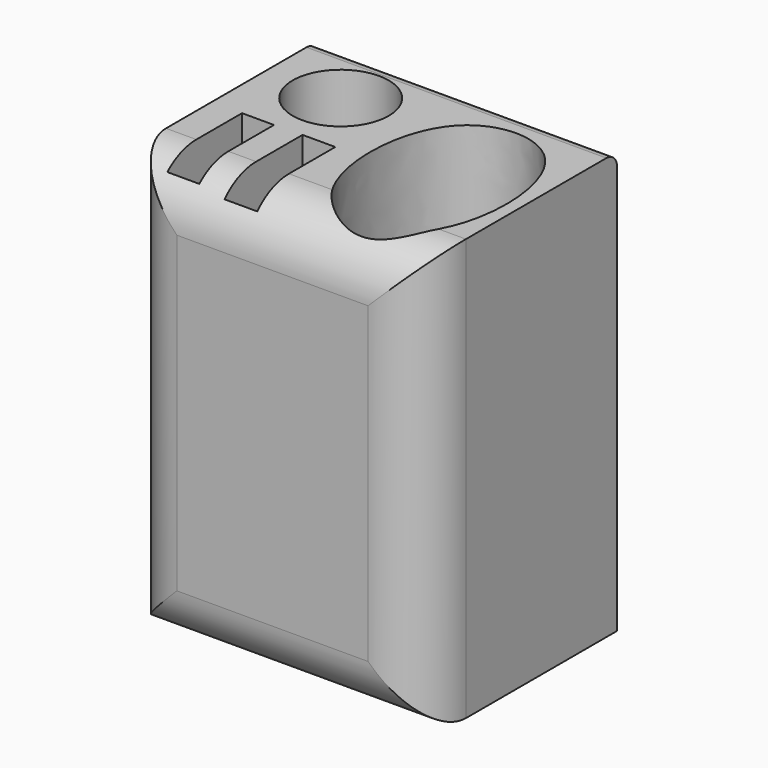
from build123d import *

# Parameters (mm, degrees)
F0_W         = 106.6799983382
F0_H         = 86.5681990981
F1_DEPTH     = 150
F6_DEPTH     = 129
F2_R         = 17.0780712093
F7_DEPTH     = 102
F5_W         = 11.6590159014
F5_H         = 34.6855749376
F8_DEPTH     = 135
F4_W         = 11.3675408065
F4_H         = 33.2281992305
F9_DEPTH     = 142
F10_T1_DEPTH = 246.5685424949
F10_T3_DEPTH = 203.2485408331
F11_R        = 4.8284271247


# Not quite as in the source:
# - a fillet or chamfer that OpenCascade refuses, or shapes differently, is made with other operations: its cross-section is extruded or revolved along the edge and cut away or added


with BuildPart() as f1:
    # F0 (on Top) → F1 (new body)
    with BuildSketch(Plane.XY):
        Rectangle(F0_W, F0_H)
    extrude(amount=F1_DEPTH)

    # F3 (on face) → F6 (cut)
    with BuildSketch(Plane.XY.offset(150)):
        with BuildLine():
            add(Edge.make_bspline(
                [(8.1613119692, 27.2529497743), (-3.0147443048, 14.6805512394), (-2.8175450086, -36.252327606), (51.2687127956, -39.2094789539), (52.3450533609, 36.9814095435), (16.8107014154, 36.9829984189), (8.1613119692, 27.2529497743)],
                knots=[0, 0, 0, 0, 0.2815356024, 0.4975750124, 0.7821135642, 1, 1, 1, 1], degree=3))
        make_face()
    extrude(amount=-F6_DEPTH, mode=Mode.SUBTRACT)

    # F2 (on face) → F7 (cut)
    with BuildSketch(Plane.XY.offset(150)):
        with Locations((-26.815738529, 20.5490160733)):
            Circle(F2_R)
    extrude(amount=-F7_DEPTH, mode=Mode.SUBTRACT)

    # F5 (on face) → F8 (cut)
    with BuildSketch(Plane.XY.offset(150)):
        with Locations((-15.4481972568, -20.6947547849)):
            Rectangle(F5_W, F5_H)
    extrude(amount=-F8_DEPTH, mode=Mode.SUBTRACT)

    # F4 (on face) → F9 (cut)
    with BuildSketch(Plane.XY.offset(150)):
        with Locations((-36.8716400117, -20.2575422591)):
            Rectangle(F4_W, F4_H)
    extrude(amount=-F9_DEPTH, mode=Mode.SUBTRACT)

    # F10: fillet of radius 19.313708499 on 4 edges, made by hand

    # F10_s2 → F10_t1 (cut)
    with BuildSketch(Plane.XY.offset(-48.2842712475)):
        with BuildLine():
            ThreePointArc((-53.3399991691, -23.9703910501), (-47.6831449196, -37.6272452996), (-34.0262906701, -43.2840995491))
            Line((-34.0262906701, -43.2840995491), (-53.3399991691, -43.2840995491))
            Line((-53.3399991691, -43.2840995491), (-53.3399991691, -23.9703910501))
        make_face()
        with BuildLine():
            ThreePointArc((53.3399991691, -23.9703910501), (47.6831449196, -37.6272452996), (34.0262906701, -43.2840995491))
            Line((34.0262906701, -43.2840995491), (53.3399991691, -43.2840995491))
            Line((53.3399991691, -43.2840995491), (53.3399991691, -23.9703910501))
        make_face()
    extrude(amount=F10_T1_DEPTH, mode=Mode.SUBTRACT)

    # F10_s4 → F10_t3 (cut)
    with BuildSketch(Plane.YZ.offset(-101.6242704166)):
        with BuildLine():
            ThreePointArc((-23.9703910501, 0), (-37.6272452996, 5.6568542495), (-43.2840995491, 19.313708499))
            Line((-43.2840995491, 19.313708499), (-43.2840995491, 0))
            Line((-43.2840995491, 0), (-23.9703910501, 0))
        make_face()
        with BuildLine():
            ThreePointArc((-23.9703910501, 150), (-37.6272452996, 144.3431457505), (-43.2840995491, 130.686291501))
            Line((-43.2840995491, 130.686291501), (-43.2840995491, 150))
            Line((-43.2840995491, 150), (-23.9703910501, 150))
        make_face()
    extrude(amount=F10_T3_DEPTH, mode=Mode.SUBTRACT)

    # F11
    f11_edges = [f1.edges().sort_by_distance(p)[0] for p in [
        (0, 43.2841, 150),
    ]]
    fillet(f11_edges, radius=F11_R)


solid = f1.part
